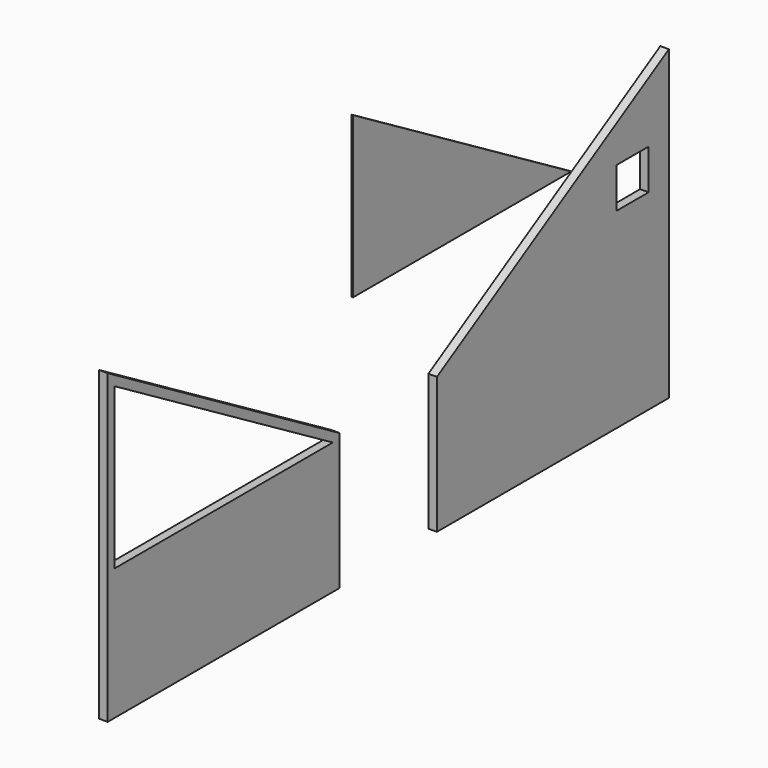
from build123d import *

# Parameters (mm, degrees)
F1_DEPTH = 12.7
F2_DEPTH = 12.7
F3_W     = 60
F3_H     = 60
F4_DEPTH = 25.4
F6_DEPTH = 2.032
F7_DEPTH = 25.4


# Not quite as in the source:
# - a length typed as a fraction of an inch, garbled in the dataset ("3 / 203.2 mm" for 3/8 in), is restored


with BuildPart() as f1:
    # F0 (on Right) → F1 (new body)
    with BuildSketch(Plane.YZ):
        Polygon((-612.9547357559, 0), (-181.1547357559, 0), (-181.1547357559, 203.2), (-612.9547357559, 457.2), align=None)
    extrude(amount=F1_DEPTH)

    # F5 (on face) → F7 (cut)
    with BuildSketch(Plane.YZ.offset(12.7)):
        Polygon((-193.8547357559, 195.9362851102), (-600.2547357559, 434.9951086396), (-600.2547357559, 195.9362851102), align=None)
    extrude(amount=-F7_DEPTH, mode=Mode.SUBTRACT)


with BuildPart() as f2:
    # F0 (on Right) → F2 (new body)
    with BuildSketch(Plane.YZ):
        Polygon((0, 203.2), (0, 0), (431.8, 0), (431.8, 457.2), align=None)
    extrude(amount=F2_DEPTH)

    # F3 (on face) → F4 (cut)
    with BuildSketch(Plane.YZ.offset(12.7)):
        with Locations((364.1244322062, 314.9529779075)):
            Rectangle(F3_W, F3_H)
    extrude(amount=-F4_DEPTH, mode=Mode.SUBTRACT)


with BuildPart() as f6:
    # F5 (on face) → F6 (new body)
    with BuildSketch(Plane.YZ.offset(12.7)):
        Polygon((247.5073088646, 372.5366592407), (-158.8926911354, 611.6014592407), (-158.8926911354, 372.5366592407), align=None)
    extrude(amount=F6_DEPTH)


solid = Compound([f1.part, f2.part, f6.part])
